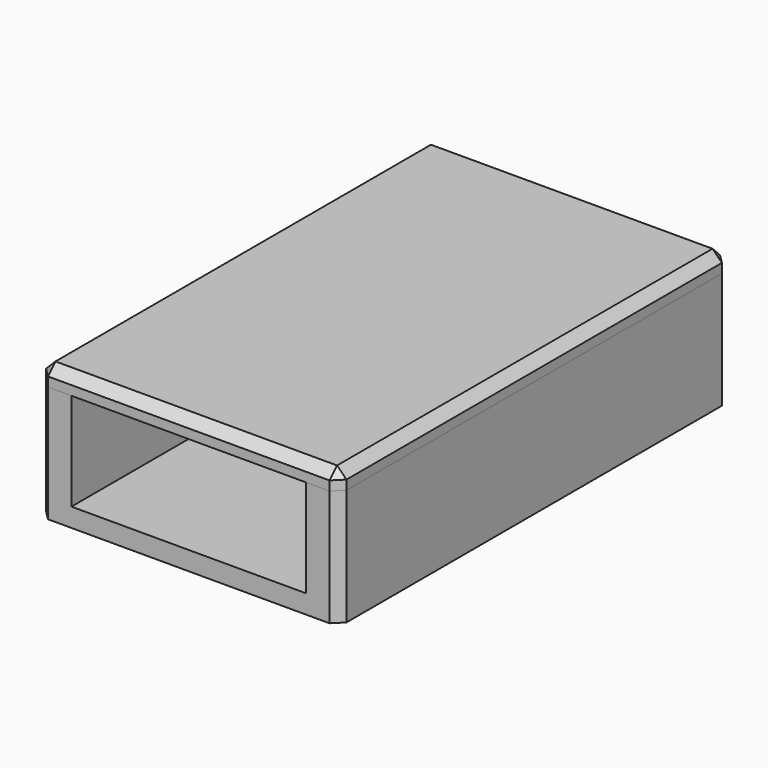
from build123d import *

# Parameters (mm, degrees)
F3_DEPTH  = 26
F1_W      = 12.5
F1_H      = 5.2
F4_DEPTH  = 1
F5_DEPTH  = 6.2
F7_DEPTH  = 1
F9_SIZE   = 0.5
F9_2_SIZE = 0.5
F10_DEPTH = 25


with BuildPart() as f3:
    # F1 (on Front) → F3 (new body)
    with BuildSketch(Plane.XZ):
        Polygon((-6.25, 1), (-6.25, 6.2), (-8, 6.2), (-8, 0), (8, 0), (8, 6.2), (6.25, 6.2), (6.25, 1), align=None)
    extrude(amount=F3_DEPTH)

    # F1 (on Front) → F4 (join)
    with BuildSketch(Plane.XZ):
        with Locations((0, 3.6)):
            Rectangle(F1_W, F1_H)
    extrude(amount=F4_DEPTH)

    # F2 (on Top) → F5 (join)
    with BuildSketch(Plane.XY):
        Polygon((-5.8, -3.15), (-6.25, -3), (-6.25, -6), (-5.8, -5.85), align=None)
        Polygon((5.8, -3.15), (5.8, -5.85), (6.25, -6), (6.25, -3), align=None)
    extrude(amount=F5_DEPTH)


with BuildPart() as f7:
    # F7 (new): a face of the model
    f7_faces = [f3.part.faces().sort_by_distance(p)[0] for p in [
        (0, -13, 0),
    ]]
    extrude(f7_faces, amount=-F7_DEPTH)


with BuildPart() as f7_1:
    # F8: moved
    add(f7.part.moved(Location((0, 0, 6.2))))

    # F9#2
    f9_2_edges = [f7_1.edges().sort_by_distance(p)[0] for p in [
        (8, -13, 7.2),
        (0, -26, 7.2),
        (-8, -13, 7.2),
        (0, 0, 7.2),
        (8, 0, 6.7),
        (8, -26, 6.7),
        (-8, -26, 6.7),
        (-8, 0, 6.7),
    ]]
    chamfer(f9_2_edges, length=F9_2_SIZE)


with BuildPart() as f3_1:
    add(f3.part)

    # F9
    f9_edges = [f3_1.edges().sort_by_distance(p)[0] for p in [
        (8, -26, 3.1),
        (-8, -26, 3.1),
        (-8, 0, 3.1),
        (8, 0, 3.1),
    ]]
    chamfer(f9_edges, length=F9_SIZE)

    # F6 (on offset) → F10 (cut)
    with BuildSketch(Plane.XY.offset(-1)):
        Polygon((-5, -2.25), (-3.2679491924, -5.25), (-1.5358983849, -2.25), align=None)
        Polygon((0, -2.25), (-1.7320508076, -5.25), (1.7320508076, -5.25), align=None)
        Polygon((3.2679491924, -5.25), (5, -2.25), (1.5358983849, -2.25), align=None)
        Polygon((-5, -9.5), (-1.5358983849, -9.5), (-3.2679491924, -6.5), align=None)
        Polygon((-1.7320508076, -6.5), (0, -9.5), (1.7320508076, -6.5), align=None)
        Polygon((3.2679491924, -6.5), (1.5358983849, -9.5), (5, -9.5), align=None)
        Polygon((5, -10.75), (1.5358983849, -10.75), (3.2679491924, -13.75), align=None)
        Polygon((0, -10.75), (-1.7320508076, -13.75), (1.7320508076, -13.75), align=None)
        Polygon((-5, -10.75), (-3.2679491924, -13.75), (-1.5358983849, -10.75), align=None)
        Polygon((-1.5358983849, -18), (-3.2679491924, -15), (-5, -18), align=None)
        Polygon((-1.7320508076, -15), (0, -18), (1.7320508076, -15), align=None)
        Polygon((3.2679491924, -15), (1.5358983849, -18), (5, -18), align=None)
    extrude(amount=F10_DEPTH, mode=Mode.SUBTRACT)


solid = Compound([f7_1.part, f3_1.part])
